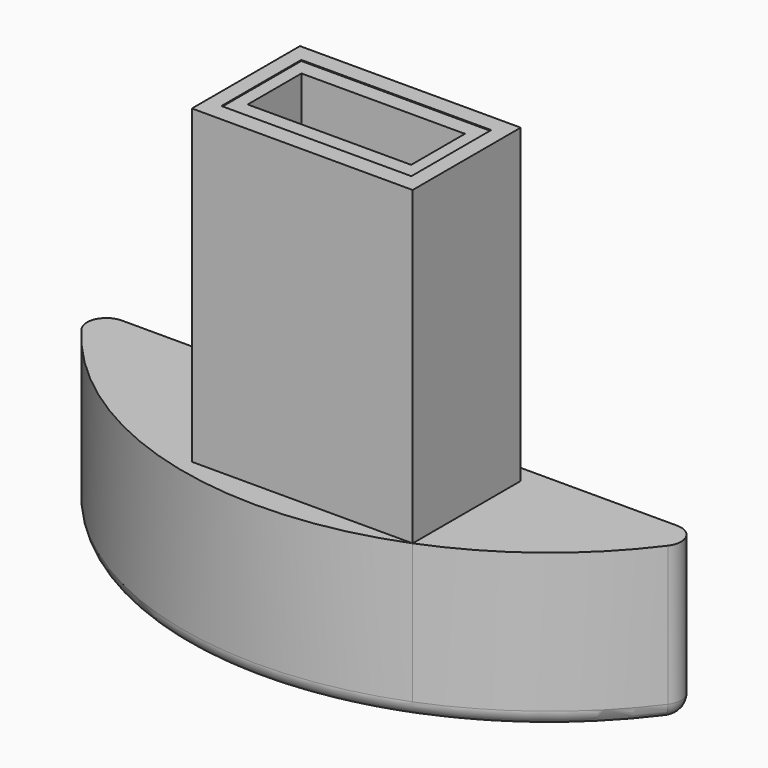
from build123d import *

# Parameters (mm, degrees)
F0_W         = 1.275
F0_H         = 0.8956698048
F0_H_2       = 0.9093301952
F0_H_3       = 0.8412417081
F1_DEPTH     = 8
F2_DEPTH     = 3
F3_DEPTH     = 21
F4_DEPTH     = 24.05
F5_R         = 1
F6_T1_DEPTH  = 28.6496073272
F6_T3_DEPTH  = 9.8
F6_T5_DEPTH  = 5.15
F6_T8_ANGLE  = 126.6295364974
F6_T10_ANGLE = 126.6295364974
F6_T12_ANGLE = 106.7409270051
F6_T17_DEPTH = 11.8
F6_T21_DEPTH = 7.15
F6_T28_DEPTH = 11.8
F6_T32_DEPTH = 7.15
F6_T39_DEPTH = 7.15
F6_T43_DEPTH = 11.8
F6_T50_DEPTH = 11.8
F6_T54_DEPTH = 7.15


# Not quite as in the source:
# - a fillet or chamfer that OpenCascade refuses, or shapes differently, is made with other operations: its cross-section is extruded or revolved along the edge and cut away or added


with BuildPart() as f1:
    # F0 (on Top) → F1 (new body)
    with BuildSketch(Plane.XY):
        with BuildLine():
            Line((0, -9.65), (-16.1925908983, -9.65))
            ThreePointArc((-16.1925908983, -9.65), (-6.0604727533, -17.8491784127), (6.9692709671, -17.5143301952))
            Line((6.9692709671, -17.5143301952), (-4.4192709671, -17.5143301952))
            Line((-4.4192709671, -17.5143301952), (-4.4192709671, -10.5456698048))
            Line((-4.4192709671, -10.5456698048), (0, -10.5456698048))
            Line((0, -10.5456698048), (0, -9.65))
        make_face()
        with BuildLine():
            ThreePointArc((6.9692709671, -17.5143301952), (12.2302855086, -14.3437309086), (16.1925908983, -9.65))
            Line((16.1925908983, -9.65), (1.275, -9.65))
            Line((1.275, -9.65), (1.275, -10.5456698048))
            Line((1.275, -10.5456698048), (6.9692709671, -10.5456698048))
            Line((6.9692709671, -10.5456698048), (6.9692709671, -17.5143301952))
        make_face()
        with Locations((0.6375, -10.0978349024)):
            Rectangle(F0_W, F0_H)
        Polygon((-4.4192709671, -17.5143301952), (6.9692709671, -17.5143301952), (6.9692709671, -10.5456698048), (1.275, -10.5456698048), (1.275, -11.455), (6.175, -11.455), (6.175, -16.605), (-3.625, -16.605), (-3.625, -11.455), (0, -11.455), (0, -10.5456698048), (-4.4192709671, -10.5456698048), align=None)
        with Locations((0.6375, -11.0003349024)):
            Rectangle(F0_W, F0_H_2)
        Polygon((0, -12.2962417081), (0, -11.455), (-3.625, -11.455), (-3.625, -16.605), (6.175, -16.605), (6.175, -11.455), (1.275, -11.455), (1.275, -12.2962417081), (5.4913964123, -12.2962417081), (5.4913964123, -15.7637582919), (-2.9413964123, -15.7637582919), (-2.9413964123, -12.2962417081), align=None)
        with Locations((0.6375, -11.875620854)):
            Rectangle(F0_W, F0_H_3)
    extrude(amount=F1_DEPTH)

    # F0 (on Top) → F2 (cut)
    with BuildSketch(Plane.XY):
        Polygon((0, -12.2962417081), (0, -11.455), (-3.625, -11.455), (-3.625, -16.605), (6.175, -16.605), (6.175, -11.455), (1.275, -11.455), (1.275, -12.2962417081), (5.4913964123, -12.2962417081), (5.4913964123, -15.7637582919), (-2.9413964123, -15.7637582919), (-2.9413964123, -12.2962417081), align=None)
        with Locations((0.6375, -11.875620854)):
            Rectangle(F0_W, F0_H_3)
    extrude(amount=F2_DEPTH, mode=Mode.SUBTRACT)

    # F3 (add): a face of the model
    f3_faces = [f1.faces().sort_by_distance(p)[0] for p in [
        (1.275, -16.4942920509, 3),
    ]]
    extrude(f3_faces, amount=-F3_DEPTH)

    # F0 (on Top) → F4 (join)
    with BuildSketch(Plane.XY):
        Polygon((-4.4192709671, -17.5143301952), (6.9692709671, -17.5143301952), (6.9692709671, -10.5456698048), (1.275, -10.5456698048), (1.275, -11.455), (6.175, -11.455), (6.175, -16.605), (-3.625, -16.605), (-3.625, -11.455), (0, -11.455), (0, -10.5456698048), (-4.4192709671, -10.5456698048), align=None)
        with Locations((0.6375, -11.0003349024)):
            Rectangle(F0_W, F0_H_2)
    extrude(amount=F4_DEPTH)

    # F5
    f5_edges = [f1.edges().sort_by_distance(p)[0] for p in [
        (16.192591, -9.65, 4),
        (-16.192591, -9.65, 4),
    ]]
    fillet(f5_edges, radius=F5_R)

    # F6: fillet of radius 0.8 on 8 edges, made by hand

    # F6_s2 → F6_t1 (cut)
    with BuildSketch(Plane.YZ.offset(-14.3248036636)):
        with BuildLine():
            ThreePointArc((-10.45, 0), (-9.8843145751, 0.2343145751), (-9.65, 0.8))
            Line((-9.65, 0.8), (-9.65, 0))
            Line((-9.65, 0), (-10.45, 0))
        make_face()
    extrude(amount=F6_T1_DEPTH, mode=Mode.SUBTRACT)

    # F6_s4 → F6_t3 (cut)
    with BuildSketch(Plane.YZ.offset(-3.625)):
        with BuildLine():
            ThreePointArc((-17.405, 0), (-16.8393145751, 0.2343145751), (-16.605, 0.8))
            Line((-16.605, 0.8), (-16.605, 0))
            Line((-16.605, 0), (-17.405, 0))
        make_face()
        with BuildLine():
            ThreePointArc((-10.655, 0), (-11.2206854249, 0.2343145751), (-11.455, 0.8))
            Line((-11.455, 0.8), (-11.455, 0))
            Line((-11.455, 0), (-10.655, 0))
        make_face()
    extrude(amount=F6_T3_DEPTH, mode=Mode.SUBTRACT)

    # F6_s6 → F6_t5 (cut)
    with BuildSketch(Plane.XZ.offset(11.455)):
        with BuildLine():
            ThreePointArc((-4.425, 0), (-3.8593145751, 0.2343145751), (-3.625, 0.8))
            Line((-3.625, 0.8), (-3.625, 0))
            Line((-3.625, 0), (-4.425, 0))
        make_face()
        with BuildLine():
            ThreePointArc((6.975, 0), (6.4093145751, 0.2343145751), (6.175, 0.8))
            Line((6.175, 0.8), (6.175, 0))
            Line((6.175, 0), (6.975, 0))
        make_face()
    extrude(amount=F6_T5_DEPTH, mode=Mode.SUBTRACT)

    # F6_s7 → F6_t8 (revolve, cut)
    with BuildSketch(Plane(origin=(0, 0, 0), x_dir=(0, 0, 1), z_dir=(-0.5966386555, -0.8025100092, 0))):
        with BuildLine():
            ThreePointArc((0, -18.05), (0.2343145751, -18.6156854249), (0.8, -18.85))
            Line((0.8, -18.85), (0, -18.85))
            Line((0, -18.85), (0, -18.05))
        make_face()
    revolve(axis=Axis((14.3248036636, -10.65, 0), (0, 0, 1)), revolution_arc=F6_T8_ANGLE, mode=Mode.SUBTRACT)

    # F6_s9 → F6_t10 (revolve, cut)
    with BuildSketch(Plane(origin=(0, 0, 0), x_dir=(0, 0, 1), z_dir=(0.5966386555, -0.8025100092, 0))):
        with BuildLine():
            ThreePointArc((0, 18.05), (0.2343145751, 18.6156854249), (0.8, 18.85))
            Line((0.8, 18.85), (0, 18.85))
            Line((0, 18.85), (0, 18.05))
        make_face()
    revolve(axis=Axis((-14.3248036636, -10.65, 0), (0, 0, -1)), revolution_arc=F6_T10_ANGLE, mode=Mode.SUBTRACT)

    # F6_s11 → F6_t12 (revolve, cut)
    with BuildSketch(Plane(origin=(0, 0, 0), x_dir=(0, 0, 1), z_dir=(-0.5966386555, 0.8025100092, 0))):
        with BuildLine():
            ThreePointArc((0.8, -18.85), (0.2343145751, -18.6156854249), (0, -18.05))
            Line((0, -18.05), (0, -18.85))
            Line((0, -18.85), (0.8, -18.85))
        make_face()
    revolve(axis=Axis((0, 0, 0), (0, 0, 1)), revolution_arc=F6_T12_ANGLE, mode=Mode.SUBTRACT)


with BuildPart() as f6_tool15:
    # F6_s16 → F6_t17 (new body)
    with BuildSketch(Plane.YZ.offset(-5.625)):
        with BuildLine():
            ThreePointArc((-17.405, 0), (-16.8393145751, 0.2343145751), (-16.605, 0.8))
            Line((-16.605, 0.8), (-16.605, 0))
            Line((-16.605, 0), (-17.405, 0))
        make_face()
    extrude(amount=F6_T17_DEPTH)

    split(bisect_by=Plane.YZ.offset(-3.625), keep=Keep.BOTTOM)


with BuildPart() as f6_tool19:
    # F6_s20 → F6_t21 (new body)
    with BuildSketch(Plane.XZ.offset(11.455)):
        with BuildLine():
            ThreePointArc((-4.425, 0), (-3.8593145751, 0.2343145751), (-3.625, 0.8))
            Line((-3.625, 0.8), (-3.625, 0))
            Line((-3.625, 0), (-4.425, 0))
        make_face()
    extrude(amount=F6_T21_DEPTH)

    split(bisect_by=Plane.XZ.offset(16.605), keep=Keep.TOP)


with BuildPart() as f6_tool15_1:
    add(f6_tool15.part)

    # F6_t23: intersect F6_tool19
    add(f6_tool19.part, mode=Mode.INTERSECT)


with BuildPart() as f1_1:
    add(f1.part)

    # F6_t13: cut F6_tool15
    add(f6_tool15_1.part, mode=Mode.SUBTRACT)


with BuildPart() as f6_tool26:
    # F6_s27 → F6_t28 (new body)
    with BuildSketch(Plane.YZ.offset(-3.625)):
        with BuildLine():
            ThreePointArc((-17.405, 0), (-16.8393145751, 0.2343145751), (-16.605, 0.8))
            Line((-16.605, 0.8), (-16.605, 0))
            Line((-16.605, 0), (-17.405, 0))
        make_face()
    extrude(amount=F6_T28_DEPTH)

    split(bisect_by=Plane.YZ.offset(6.175), keep=Keep.TOP)


with BuildPart() as f6_tool30:
    # F6_s31 → F6_t32 (new body)
    with BuildSketch(Plane.XZ.offset(18.605)):
        with BuildLine():
            ThreePointArc((6.975, 0), (6.4093145751, 0.2343145751), (6.175, 0.8))
            Line((6.175, 0.8), (6.175, 0))
            Line((6.175, 0), (6.975, 0))
        make_face()
    extrude(amount=-F6_T32_DEPTH)

    split(bisect_by=Plane.XZ.offset(16.605), keep=Keep.TOP)


with BuildPart() as f6_tool26_1:
    add(f6_tool26.part)

    # F6_t34: intersect F6_tool30
    add(f6_tool30.part, mode=Mode.INTERSECT)


with BuildPart() as f1_2:
    add(f1_1.part)

    # F6_t24: cut F6_tool26
    add(f6_tool26_1.part, mode=Mode.SUBTRACT)


with BuildPart() as f6_tool37:
    # F6_s38 → F6_t39 (new body)
    with BuildSketch(Plane.XZ.offset(9.455)):
        with BuildLine():
            ThreePointArc((-4.425, 0), (-3.8593145751, 0.2343145751), (-3.625, 0.8))
            Line((-3.625, 0.8), (-3.625, 0))
            Line((-3.625, 0), (-4.425, 0))
        make_face()
    extrude(amount=F6_T39_DEPTH)

    split(bisect_by=Plane.XZ.offset(11.455), keep=Keep.BOTTOM)


with BuildPart() as f6_tool41:
    # F6_s42 → F6_t43 (new body)
    with BuildSketch(Plane.YZ.offset(6.175)):
        with BuildLine():
            ThreePointArc((-10.655, 0), (-11.2206854249, 0.2343145751), (-11.455, 0.8))
            Line((-11.455, 0.8), (-11.455, 0))
            Line((-11.455, 0), (-10.655, 0))
        make_face()
    extrude(amount=-F6_T43_DEPTH)

    split(bisect_by=Plane.YZ.offset(-3.625), keep=Keep.BOTTOM)


with BuildPart() as f6_tool37_1:
    add(f6_tool37.part)

    # F6_t45: intersect F6_tool41
    add(f6_tool41.part, mode=Mode.INTERSECT)


with BuildPart() as f1_3:
    add(f1_2.part)

    # F6_t35: cut F6_tool37
    add(f6_tool37_1.part, mode=Mode.SUBTRACT)


with BuildPart() as f6_tool48:
    # F6_s49 → F6_t50 (new body)
    with BuildSketch(Plane.YZ.offset(8.175)):
        with BuildLine():
            ThreePointArc((-10.655, 0), (-11.2206854249, 0.2343145751), (-11.455, 0.8))
            Line((-11.455, 0.8), (-11.455, 0))
            Line((-11.455, 0), (-10.655, 0))
        make_face()
    extrude(amount=-F6_T50_DEPTH)

    split(bisect_by=Plane.YZ.offset(6.175), keep=Keep.TOP)


with BuildPart() as f6_tool52:
    # F6_s53 → F6_t54 (new body)
    with BuildSketch(Plane.XZ.offset(16.605)):
        with BuildLine():
            ThreePointArc((6.975, 0), (6.4093145751, 0.2343145751), (6.175, 0.8))
            Line((6.175, 0.8), (6.175, 0))
            Line((6.175, 0), (6.975, 0))
        make_face()
    extrude(amount=-F6_T54_DEPTH)

    split(bisect_by=Plane.XZ.offset(11.455), keep=Keep.BOTTOM)


with BuildPart() as f6_tool48_1:
    add(f6_tool48.part)

    # F6_t56: intersect F6_tool52
    add(f6_tool52.part, mode=Mode.INTERSECT)


with BuildPart() as f1_4:
    add(f1_3.part)

    # F6_t46: cut F6_tool48
    add(f6_tool48_1.part, mode=Mode.SUBTRACT)


solid = f1_4.part
